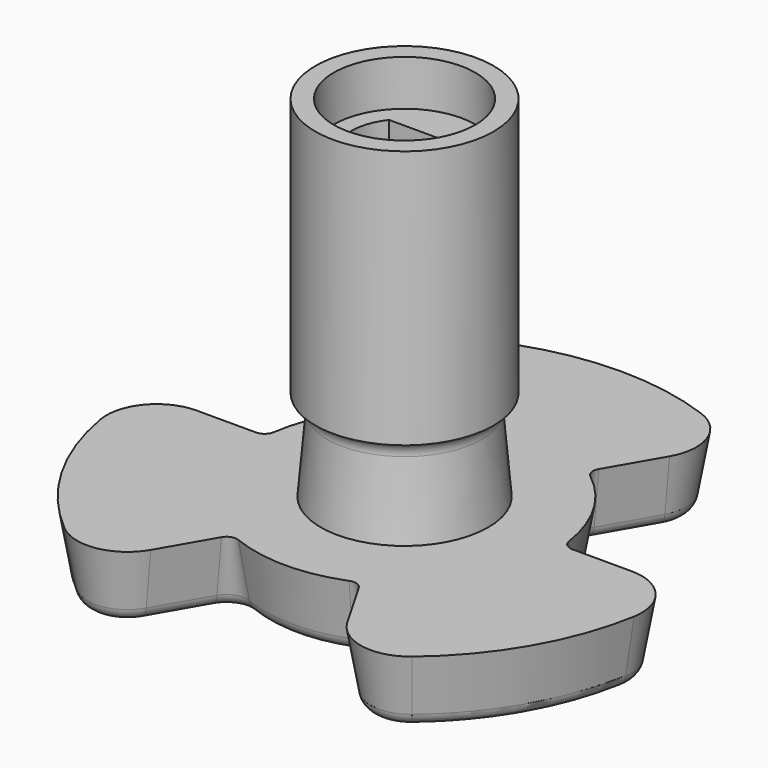
from build123d import *

# Parameters (mm, degrees)
F1_DEPTH     = 4.5
F1_TAPER     = -10
F2_R         = 5.5
F3_DEPTH     = 6
F3_TAPER     = 5
F4_R         = 5.85
F5_DEPTH     = 17
F6_T5_DEPTH  = 3.8905520117
F6_T8_ANGLE  = 99.9281918423
F6_T11_ANGLE = 81.7867892983
F6_T14_ANGLE = 40.1436163154
F6_T17_ANGLE = 43.5735785965
F6_T20_ANGLE = 99.9281918423
F6_T23_ANGLE = 81.7867892983
F6_T26_DEPTH = 3.8905520117
F6_T29_DEPTH = 3.8905520117
F6_T32_ANGLE = 81.7867892983
F6_T35_ANGLE = 99.9281918423
F6_T38_ANGLE = 43.5735785965
F6_T41_ANGLE = 40.1436163154
F6_T44_ANGLE = 81.7867892983
F6_T47_ANGLE = 99.9281918423
F6_T50_DEPTH = 3.8905520117
F6_T53_DEPTH = 3.8905520117
F6_T56_ANGLE = 99.9281918423
F6_T59_ANGLE = 81.7867892983
F6_T62_ANGLE = 40.1436163154
F6_T65_ANGLE = 43.5735785965
F6_T68_ANGLE = 99.9281918423
F6_T71_ANGLE = 81.7867892983
F6_T74_DEPTH = 3.8905520117
F7_R         = 4.65
F8_DEPTH     = 3
F10_DEPTH    = 21.5
F11_R        = 2
F12_DEPTH    = 1.5


# Not quite as in the source:
# - a fillet or chamfer that OpenCascade refuses, or shapes differently, is made with other operations: its cross-section is extruded or revolved along the edge and cut away or added


with BuildPart() as f1:
    # F0 (on Top) → F1 (new body)
    with BuildSketch(Plane.XY):
        with BuildLine():
            ThreePointArc((-14.2828568571, 0), (-16.1969605908, -0.8918311977), (-16.7454183842, -2.9310344828))
            ThreePointArc((-16.7454183842, -2.9310344828), (-14.7224318643, -8.5), (-10.9110595135, -13.0364404763))
            ThreePointArc((-10.9110595135, -13.0364404763), (-8.8708287685, -13.5810637369), (-7.1414284285, -12.3693168769))
            Line((-7.1414284285, -12.3693168769), (-5.1961524227, -9))
            ThreePointArc((-5.1961524227, -9), (-4.3881045701, -8.3326332262), (-3.3403837003, -8.3571428571))
            ThreePointArc((-3.3403837003, -8.3571428571), (0, -9), (3.3403837003, -8.3571428571))
            ThreePointArc((3.3403837003, -8.3571428571), (4.3881045701, -8.3326332262), (5.1961524227, -9))
            Line((5.1961524227, -9), (7.1414284285, -12.3693168769))
            ThreePointArc((7.1414284285, -12.3693168769), (8.8708287685, -13.5810637369), (10.9110595135, -13.0364404763))
            ThreePointArc((10.9110595135, -13.0364404763), (14.7224318643, -8.5), (16.7454183842, -2.9310344828))
            ThreePointArc((16.7454183842, -2.9310344828), (16.1969605908, -0.8918311977), (14.2828568571, 0))
            Line((14.2828568571, 0), (10.3923048454, 0))
            ThreePointArc((10.3923048454, 0), (9.4103243394, 0.366106581), (8.9076898675, 1.2857142857))
            ThreePointArc((8.9076898675, 1.2857142857), (7.7942286341, 4.5), (5.5673061672, 7.0714285714))
            ThreePointArc((5.5673061672, 7.0714285714), (5.0222197693, 7.9665266452), (5.1961524227, 9))
            Line((5.1961524227, 9), (7.1414284285, 12.3693168769))
            ThreePointArc((7.1414284285, 12.3693168769), (7.3261318223, 14.4728949346), (5.8343588706, 15.9674749591))
            ThreePointArc((5.8343588706, 15.9674749591), (0, 17), (-5.8343588706, 15.9674749591))
            ThreePointArc((-5.8343588706, 15.9674749591), (-7.3261318223, 14.4728949346), (-7.1414284285, 12.3693168769))
            Line((-7.1414284285, 12.3693168769), (-5.1961524227, 9))
            ThreePointArc((-5.1961524227, 9), (-5.0222197693, 7.9665266452), (-5.5673061672, 7.0714285714))
            ThreePointArc((-5.5673061672, 7.0714285714), (-7.7942286341, 4.5), (-8.9076898675, 1.2857142857))
            ThreePointArc((-8.9076898675, 1.2857142857), (-9.4103243394, 0.366106581), (-10.3923048454, 0))
            Line((-10.3923048454, 0), (-14.2828568571, 0))
        make_face()
    extrude(amount=F1_DEPTH, taper=F1_TAPER)

    # F2 (on face) → F3 (join)
    with BuildSketch(Plane.XY.offset(4.5)):
        Circle(F2_R)
    extrude(amount=F3_DEPTH, taper=F3_TAPER)

    # F4 (on face) → F5 (join)
    with BuildSketch(Plane.XY.offset(10.5)):
        Circle(F4_R)
    extrude(amount=F5_DEPTH)

    # F6: fillet of radius 1 on 25 edges, made by hand

    # F6_s1 → F6_t2 (revolve)
    with BuildSketch(Plane.XZ):
        with BuildLine():
            ThreePointArc((5.85, 10.5), (5.2585337353, 10.115416547), (5.0681484473, 9.4360858347))
            Line((5.0681484473, 9.4360858347), (5.0482245533, 9.4343427198))
            Line((5.0482245533, 9.4343427198), (4.9551441249, 10.4982568851))
            Line((4.9551441249, 10.4982568851), (4.9750680188, 10.52))
            ThreePointArc((4.9750680188, 10.52), (5.4125340094, 10.52), (5.8457131371, 10.5195351685))
            Line((5.8457131371, 10.5195351685), (5.85, 10.5))
        make_face()
    revolve(axis=Axis((0, 0, 10.5), (0, 0, -1)))


with BuildPart() as f6_tool3:
    # F6_s4 → F6_t5 (new body)
    with BuildSketch(Plane(origin=(-7.1414284285, 12.3693168769, 0), x_dir=(0, 0, 1), z_dir=(0.5, -0.8660254038, 0))):
        with BuildLine():
            ThreePointArc((0.8263518223, 0.1457081218), (0.2339555569, -0.1963120215), (0, -0.8390996312))
            Line((0, -0.8390996312), (-0.02, -0.8390996312))
            Line((-0.02, -0.8390996312), (-0.02, 0.0167819926))
            Line((-0.02, 0.0167819926), (0.8228788588, 0.1654042769))
            Line((0.8228788588, 0.1654042769), (0.8263518223, 0.1457081218))
        make_face()
    extrude(amount=F6_T5_DEPTH)


with BuildPart() as f6_tool6:
    # F6_s7 → F6_t8 (revolve)
    with BuildSketch(Plane(origin=(0, 0, 0), x_dir=(0, 0, 1), z_dir=(0.9392632329, 0.3431975806, 0))):
        with BuildLine():
            ThreePointArc((0.8263518223, -17.1457081218), (0.2339555569, -16.8036879785), (0, -16.1609003688))
            Line((0, -16.1609003688), (-0.02, -16.1609003688))
            Line((-0.02, -16.1609003688), (-0.02, -17.0167819926))
            Line((-0.02, -17.0167819926), (0.8228788588, -17.1654042769))
            Line((0.8228788588, -17.1654042769), (0.8263518223, -17.1457081218))
        make_face()
    revolve(axis=Axis((-4.9763649191, 13.6193168769, 0), (0, 0, 1)), revolution_arc=F6_T8_ANGLE)


with BuildPart() as f6_tool9:
    # F6_s10 → F6_t11 (revolve)
    with BuildSketch(Plane(origin=(-5.1961524227, 9, 0), x_dir=(0, 0, 1), z_dir=(-0.5, 0.8660254038, 0))):
        with BuildLine():
            ThreePointArc((0.8263518223, -0.1457081218), (0.2339555569, 0.1963120215), (0, 0.8390996312))
            Line((0, 0.8390996312), (-0.02, 0.8390996312))
            Line((-0.02, 0.8390996312), (-0.02, -0.0167819926))
            Line((-0.02, -0.0167819926), (0.8228788588, -0.1654042769))
            Line((0.8228788588, -0.1654042769), (0.8263518223, -0.1457081218))
        make_face()
    revolve(axis=Axis((-6.4951905284, 8.25, 0), (0, 0, -1)), revolution_arc=F6_T11_ANGLE)


with BuildPart() as f6_tool12:
    # F6_s13 → F6_t14 (revolve)
    with BuildSketch(Plane(origin=(0, 0, 0), x_dir=(0, 0, 1), z_dir=(0.9392632329, -0.3431975806, 0))):
        with BuildLine():
            ThreePointArc((0.8263518223, -17.1457081218), (0.2339555569, -16.8036879785), (0, -16.1609003688))
            Line((0, -16.1609003688), (-0.02, -16.1609003688))
            Line((-0.02, -16.1609003688), (-0.02, -17.0167819926))
            Line((-0.02, -17.0167819926), (0.8228788588, -17.1654042769))
            Line((0.8228788588, -17.1654042769), (0.8263518223, -17.1457081218))
        make_face()
    revolve(axis=Axis((0, 0, 0), (0, 0, 1)), revolution_arc=F6_T14_ANGLE)


with BuildPart() as f6_tool15:
    # F6_s16 → F6_t17 (revolve)
    with BuildSketch(Plane(origin=(0, 0, 0), x_dir=(0, 0, 1), z_dir=(0.7857142857, 0.6185895741, 0))):
        with BuildLine():
            ThreePointArc((0.8263518223, -9.1457081218), (0.2339555569, -8.8036879785), (0, -8.1609003688))
            Line((0, -8.1609003688), (-0.02, -8.1609003688))
            Line((-0.02, -8.1609003688), (-0.02, -9.0167819926))
            Line((-0.02, -9.0167819926), (0.8228788588, -9.1654042769))
            Line((0.8228788588, -9.1654042769), (0.8263518223, -9.1457081218))
        make_face()
    revolve(axis=Axis((0, 0, 0), (0, 0, 1)), revolution_arc=F6_T17_ANGLE)


with BuildPart() as f6_tool18:
    # F6_s19 → F6_t20 (revolve)
    with BuildSketch(Plane(origin=(7.1414284285, 12.3693168769, 0), x_dir=(0, 0, 1), z_dir=(-0.5, -0.8660254038, 0))):
        with BuildLine():
            ThreePointArc((0.8263518223, -0.1457081218), (0.2339555569, 0.1963120215), (0, 0.8390996312))
            Line((0, 0.8390996312), (-0.02, 0.8390996312))
            Line((-0.02, 0.8390996312), (-0.02, -0.0167819926))
            Line((-0.02, -0.0167819926), (0.8228788588, -0.1654042769))
            Line((0.8228788588, -0.1654042769), (0.8263518223, -0.1457081218))
        make_face()
    revolve(axis=Axis((4.9763649191, 13.6193168769, 0), (0, 0, 1)), revolution_arc=F6_T20_ANGLE)


with BuildPart() as f6_tool21:
    # F6_s22 → F6_t23 (revolve)
    with BuildSketch(Plane(origin=(0, 0, 0), x_dir=(0, 0, 1), z_dir=(0.1428571429, 0.9897433186, 0))):
        with BuildLine():
            ThreePointArc((0.8263518223, -9.1457081218), (0.2339555569, -8.8036879785), (0, -8.1609003688))
            Line((0, -8.1609003688), (-0.02, -8.1609003688))
            Line((-0.02, -8.1609003688), (-0.02, -9.0167819926))
            Line((-0.02, -9.0167819926), (0.8228788588, -9.1654042769))
            Line((0.8228788588, -9.1654042769), (0.8263518223, -9.1457081218))
        make_face()
    revolve(axis=Axis((-10.3923048454, 1.5, 0), (0, 0, -1)), revolution_arc=F6_T23_ANGLE)


with BuildPart() as f6_tool24:
    # F6_s25 → F6_t26 (new body)
    with BuildSketch(Plane(origin=(5.1961524227, 9, 0), x_dir=(0, 0, 1), z_dir=(0.5, 0.8660254038, 0))):
        with BuildLine():
            ThreePointArc((0.8263518223, 0.1457081218), (0.2339555569, -0.1963120215), (0, -0.8390996312))
            Line((0, -0.8390996312), (-0.02, -0.8390996312))
            Line((-0.02, -0.8390996312), (-0.02, 0.0167819926))
            Line((-0.02, 0.0167819926), (0.8228788588, 0.1654042769))
            Line((0.8228788588, 0.1654042769), (0.8263518223, 0.1457081218))
        make_face()
    extrude(amount=F6_T26_DEPTH)


with BuildPart() as f6_tool27:
    # F6_s28 → F6_t29 (new body)
    with BuildSketch(Plane.YZ.offset(-10.3923048454)):
        with BuildLine():
            ThreePointArc((0.1457081218, 0.8263518223), (-0.1963120215, 0.2339555569), (-0.8390996312, 0))
            Line((-0.8390996312, 0), (-0.8390996312, -0.02))
            Line((-0.8390996312, -0.02), (0.0167819926, -0.02))
            Line((0.0167819926, -0.02), (0.1654042769, 0.8228788588))
            Line((0.1654042769, 0.8228788588), (0.1457081218, 0.8263518223))
        make_face()
    extrude(amount=-F6_T29_DEPTH)


with BuildPart() as f6_tool30:
    # F6_s31 → F6_t32 (revolve)
    with BuildSketch(Plane(origin=(0, 0, 0), x_dir=(0, 0, 1), z_dir=(0.7857142857, -0.6185895741, 0))):
        with BuildLine():
            ThreePointArc((0.8263518223, -9.1457081218), (0.2339555569, -8.8036879785), (0, -8.1609003688))
            Line((0, -8.1609003688), (-0.02, -8.1609003688))
            Line((-0.02, -8.1609003688), (-0.02, -9.0167819926))
            Line((-0.02, -9.0167819926), (0.8228788588, -9.1654042769))
            Line((0.8228788588, -9.1654042769), (0.8263518223, -9.1457081218))
        make_face()
    revolve(axis=Axis((6.4951905284, 8.25, 0), (0, 0, -1)), revolution_arc=F6_T32_ANGLE)


with BuildPart() as f6_tool33:
    # F6_s34 → F6_t35 (revolve)
    with BuildSketch(Plane.YZ.offset(-14.2828568571)):
        with BuildLine():
            ThreePointArc((0.1457081218, 0.8263518223), (-0.1963120215, 0.2339555569), (-0.8390996312, 0))
            Line((-0.8390996312, 0), (-0.8390996312, -0.02))
            Line((-0.8390996312, -0.02), (0.0167819926, -0.02))
            Line((0.0167819926, -0.02), (0.1654042769, 0.8228788588))
            Line((0.1654042769, 0.8228788588), (0.1457081218, 0.8263518223))
        make_face()
    revolve(axis=Axis((-14.2828568571, -2.5, 0), (0, 0, 1)), revolution_arc=F6_T35_ANGLE)


with BuildPart() as f6_tool36:
    # F6_s37 → F6_t38 (revolve)
    with BuildSketch(Plane(origin=(0, 0, 0), x_dir=(0, 0, 1), z_dir=(0.1428571429, -0.9897433186, 0))):
        with BuildLine():
            ThreePointArc((0.8263518223, -9.1457081218), (0.2339555569, -8.8036879785), (0, -8.1609003688))
            Line((0, -8.1609003688), (-0.02, -8.1609003688))
            Line((-0.02, -8.1609003688), (-0.02, -9.0167819926))
            Line((-0.02, -9.0167819926), (0.8228788588, -9.1654042769))
            Line((0.8228788588, -9.1654042769), (0.8263518223, -9.1457081218))
        make_face()
    revolve(axis=Axis((0, 0, 0), (0, 0, 1)), revolution_arc=F6_T38_ANGLE)


with BuildPart() as f6_tool39:
    # F6_s40 → F6_t41 (revolve)
    with BuildSketch(Plane(origin=(0, 0, 0), x_dir=(0, 0, 1), z_dir=(-0.1724137931, 0.9850246108, 0))):
        with BuildLine():
            ThreePointArc((0.8263518223, -17.1457081218), (0.2339555569, -16.8036879785), (0, -16.1609003688))
            Line((0, -16.1609003688), (-0.02, -16.1609003688))
            Line((-0.02, -16.1609003688), (-0.02, -17.0167819926))
            Line((-0.02, -17.0167819926), (0.8228788588, -17.1654042769))
            Line((0.8228788588, -17.1654042769), (0.8263518223, -17.1457081218))
        make_face()
    revolve(axis=Axis((0, 0, 0), (0, 0, 1)), revolution_arc=F6_T41_ANGLE)


with BuildPart() as f6_tool42:
    # F6_s43 → F6_t44 (revolve)
    with BuildSketch(Plane.YZ.offset(10.3923048454)):
        with BuildLine():
            ThreePointArc((0.1457081218, 0.8263518223), (-0.1963120215, 0.2339555569), (-0.8390996312, 0))
            Line((-0.8390996312, 0), (-0.8390996312, -0.02))
            Line((-0.8390996312, -0.02), (0.0167819926, -0.02))
            Line((0.0167819926, -0.02), (0.1654042769, 0.8228788588))
            Line((0.1654042769, 0.8228788588), (0.1457081218, 0.8263518223))
        make_face()
    revolve(axis=Axis((10.3923048454, 1.5, 0), (0, 0, -1)), revolution_arc=F6_T44_ANGLE)


with BuildPart() as f6_tool45:
    # F6_s46 → F6_t47 (revolve)
    with BuildSketch(Plane(origin=(0, 0, 0), x_dir=(0, 0, 1), z_dir=(-0.7668494398, 0.6418270302, 0))):
        with BuildLine():
            ThreePointArc((0.8263518223, -17.1457081218), (0.2339555569, -16.8036879785), (0, -16.1609003688))
            Line((0, -16.1609003688), (-0.02, -16.1609003688))
            Line((-0.02, -16.1609003688), (-0.02, -17.0167819926))
            Line((-0.02, -17.0167819926), (0.8228788588, -17.1654042769))
            Line((0.8228788588, -17.1654042769), (0.8263518223, -17.1457081218))
        make_face()
    revolve(axis=Axis((-9.306491938, -11.1193168769, 0), (0, 0, 1)), revolution_arc=F6_T47_ANGLE)


with BuildPart() as f6_tool48:
    # F6_s49 → F6_t50 (new body)
    with BuildSketch(Plane.YZ.offset(14.2828568571)):
        with BuildLine():
            ThreePointArc((0.1457081218, 0.8263518223), (-0.1963120215, 0.2339555569), (-0.8390996312, 0))
            Line((-0.8390996312, 0), (-0.8390996312, -0.02))
            Line((-0.8390996312, -0.02), (0.0167819926, -0.02))
            Line((0.0167819926, -0.02), (0.1654042769, 0.8228788588))
            Line((0.1654042769, 0.8228788588), (0.1457081218, 0.8263518223))
        make_face()
    extrude(amount=-F6_T50_DEPTH)


with BuildPart() as f6_tool51:
    # F6_s52 → F6_t53 (new body)
    with BuildSketch(Plane(origin=(-7.1414284285, -12.3693168769, 0), x_dir=(0, 0, 1), z_dir=(0.5, 0.8660254038, 0))):
        with BuildLine():
            ThreePointArc((0.8263518223, 0.1457081218), (0.2339555569, -0.1963120215), (0, -0.8390996312))
            Line((0, -0.8390996312), (-0.02, -0.8390996312))
            Line((-0.02, -0.8390996312), (-0.02, 0.0167819926))
            Line((-0.02, 0.0167819926), (0.8228788588, 0.1654042769))
            Line((0.8228788588, 0.1654042769), (0.8263518223, 0.1457081218))
        make_face()
    extrude(amount=F6_T53_DEPTH)


with BuildPart() as f6_tool54:
    # F6_s55 → F6_t56 (revolve)
    with BuildSketch(Plane(origin=(0, 0, 0), x_dir=(0, 0, 1), z_dir=(-0.1724137931, -0.9850246108, 0))):
        with BuildLine():
            ThreePointArc((0.8263518223, -17.1457081218), (0.2339555569, -16.8036879785), (0, -16.1609003688))
            Line((0, -16.1609003688), (-0.02, -16.1609003688))
            Line((-0.02, -16.1609003688), (-0.02, -17.0167819926))
            Line((-0.02, -17.0167819926), (0.8228788588, -17.1654042769))
            Line((0.8228788588, -17.1654042769), (0.8263518223, -17.1457081218))
        make_face()
    revolve(axis=Axis((14.2828568571, -2.5, 0), (0, 0, 1)), revolution_arc=F6_T56_ANGLE)


with BuildPart() as f6_tool57:
    # F6_s58 → F6_t59 (revolve)
    with BuildSketch(Plane(origin=(-5.1961524227, -9, 0), x_dir=(0, 0, 1), z_dir=(-0.5, -0.8660254038, 0))):
        with BuildLine():
            ThreePointArc((0.8263518223, -0.1457081218), (0.2339555569, 0.1963120215), (0, 0.8390996312))
            Line((0, 0.8390996312), (-0.02, 0.8390996312))
            Line((-0.02, 0.8390996312), (-0.02, -0.0167819926))
            Line((-0.02, -0.0167819926), (0.8228788588, -0.1654042769))
            Line((0.8228788588, -0.1654042769), (0.8263518223, -0.1457081218))
        make_face()
    revolve(axis=Axis((-3.897114317, -9.75, 0), (0, 0, -1)), revolution_arc=F6_T59_ANGLE)


with BuildPart() as f6_tool60:
    # F6_s61 → F6_t62 (revolve)
    with BuildSketch(Plane(origin=(0, 0, 0), x_dir=(0, 0, 1), z_dir=(-0.7668494398, -0.6418270302, 0))):
        with BuildLine():
            ThreePointArc((0.8263518223, -17.1457081218), (0.2339555569, -16.8036879785), (0, -16.1609003688))
            Line((0, -16.1609003688), (-0.02, -16.1609003688))
            Line((-0.02, -16.1609003688), (-0.02, -17.0167819926))
            Line((-0.02, -17.0167819926), (0.8228788588, -17.1654042769))
            Line((0.8228788588, -17.1654042769), (0.8263518223, -17.1457081218))
        make_face()
    revolve(axis=Axis((0, 0, 0), (0, 0, 1)), revolution_arc=F6_T62_ANGLE)


with BuildPart() as f6_tool63:
    # F6_s64 → F6_t65 (revolve)
    with BuildSketch(Plane(origin=(0, 0, 0), x_dir=(0, 0, 1), z_dir=(-0.9285714286, 0.3711537445, 0))):
        with BuildLine():
            ThreePointArc((0.8263518223, -9.1457081218), (0.2339555569, -8.8036879785), (0, -8.1609003688))
            Line((0, -8.1609003688), (-0.02, -8.1609003688))
            Line((-0.02, -8.1609003688), (-0.02, -9.0167819926))
            Line((-0.02, -9.0167819926), (0.8228788588, -9.1654042769))
            Line((0.8228788588, -9.1654042769), (0.8263518223, -9.1457081218))
        make_face()
    revolve(axis=Axis((0, 0, 0), (0, 0, 1)), revolution_arc=F6_T65_ANGLE)


with BuildPart() as f6_tool66:
    # F6_s67 → F6_t68 (revolve)
    with BuildSketch(Plane(origin=(7.1414284285, -12.3693168769, 0), x_dir=(0, 0, 1), z_dir=(-0.5, 0.8660254038, 0))):
        with BuildLine():
            ThreePointArc((0.8263518223, -0.1457081218), (0.2339555569, 0.1963120215), (0, 0.8390996312))
            Line((0, 0.8390996312), (-0.02, 0.8390996312))
            Line((-0.02, 0.8390996312), (-0.02, -0.0167819926))
            Line((-0.02, -0.0167819926), (0.8228788588, -0.1654042769))
            Line((0.8228788588, -0.1654042769), (0.8263518223, -0.1457081218))
        make_face()
    revolve(axis=Axis((9.306491938, -11.1193168769, 0), (0, 0, 1)), revolution_arc=F6_T68_ANGLE)


with BuildPart() as f6_tool69:
    # F6_s70 → F6_t71 (revolve)
    with BuildSketch(Plane(origin=(0, 0, 0), x_dir=(0, 0, 1), z_dir=(-0.9285714286, -0.3711537445, 0))):
        with BuildLine():
            ThreePointArc((0.8263518223, -9.1457081218), (0.2339555569, -8.8036879785), (0, -8.1609003688))
            Line((0, -8.1609003688), (-0.02, -8.1609003688))
            Line((-0.02, -8.1609003688), (-0.02, -9.0167819926))
            Line((-0.02, -9.0167819926), (0.8228788588, -9.1654042769))
            Line((0.8228788588, -9.1654042769), (0.8263518223, -9.1457081218))
        make_face()
    revolve(axis=Axis((3.897114317, -9.75, 0), (0, 0, -1)), revolution_arc=F6_T71_ANGLE)


with BuildPart() as f6_tool72:
    # F6_s73 → F6_t74 (new body)
    with BuildSketch(Plane(origin=(5.1961524227, -9, 0), x_dir=(0, 0, 1), z_dir=(0.5, -0.8660254038, 0))):
        with BuildLine():
            ThreePointArc((0.8263518223, 0.1457081218), (0.2339555569, -0.1963120215), (0, -0.8390996312))
            Line((0, -0.8390996312), (-0.02, -0.8390996312))
            Line((-0.02, -0.8390996312), (-0.02, 0.0167819926))
            Line((-0.02, 0.0167819926), (0.8228788588, 0.1654042769))
            Line((0.8228788588, 0.1654042769), (0.8263518223, 0.1457081218))
        make_face()
    extrude(amount=F6_T74_DEPTH)


with BuildPart() as f1_1:
    add(f1.part)

    # F6_t75: cut F6_tool3, F6_tool6, F6_tool9, F6_tool12, F6_tool15, F6_tool18, F6_tool21, F6_tool24, F6_tool27, F6_tool30, F6_tool33, F6_tool36, F6_tool39, F6_tool42, F6_tool45, F6_tool48, F6_tool51, F6_tool54, F6_tool57, F6_tool60, F6_tool63, F6_tool66, F6_tool69, F6_tool72
    add([f6_tool3.part, f6_tool6.part, f6_tool9.part, f6_tool12.part, f6_tool15.part, f6_tool18.part, f6_tool21.part, f6_tool24.part, f6_tool27.part, f6_tool30.part, f6_tool33.part, f6_tool36.part, f6_tool39.part, f6_tool42.part, f6_tool45.part, f6_tool48.part, f6_tool51.part, f6_tool54.part, f6_tool57.part, f6_tool60.part, f6_tool63.part, f6_tool66.part, f6_tool69.part, f6_tool72.part], mode=Mode.SUBTRACT)

    # F7 (on face) → F8 (cut)
    with BuildSketch(Plane.XY.offset(27.5)):
        Circle(F7_R)
    extrude(amount=-F8_DEPTH, mode=Mode.SUBTRACT)

    # F9 (on face) → F10 (cut)
    with BuildSketch(Plane.XY.offset(24.5)):
        with BuildLine():
            Line((2.75, 2.1650635095), (-2.75, 2.1650635095))
            ThreePointArc((-2.75, 2.1650635095), (-3.5, 0), (-2.75, -2.1650635095))
            Line((-2.75, -2.1650635095), (2.75, -2.1650635095))
            ThreePointArc((2.75, -2.1650635095), (3.5, 0), (2.75, 2.1650635095))
        make_face()
    extrude(amount=-F10_DEPTH, mode=Mode.SUBTRACT)

    # F11 (on face) → F12 (cut)
    with BuildSketch(Plane(origin=(0, 0, 0), x_dir=(1, 0, 0), z_dir=(0, 0, -1))):
        Circle(F11_R)
    extrude(amount=-F12_DEPTH, mode=Mode.SUBTRACT)


solid = f1_1.part
